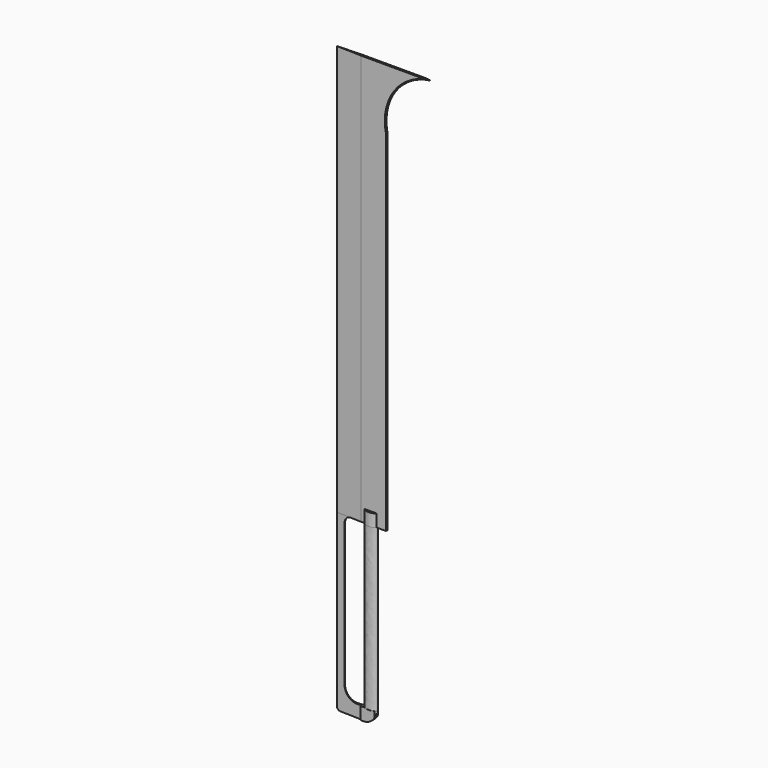
from build123d import *

# Parameters (mm, degrees)
F0_W          = 101.6
F0_H          = 838.2
F1_DEPTH      = 1.905
F3_DEPTH      = 330.2
F3_DEPTH_BACK = 25.4
F5_DEPTH      = 838.201
F7_DEPTH      = 1.905
F9_DEPTH      = 3.96875
F11_DEPTH     = 355.6010001
F13_DEPTH     = 25.401
F14_T2_ANGLE  = 126.8514429449
F14_T4_ANGLE  = 126.8514429449


# Not quite as in the source:
# - a fillet or chamfer that OpenCascade refuses, or shapes differently, is made with other operations: its cross-section is extruded or revolved along the edge and cut away or added


with BuildPart() as f1:
    # F0 (on Front) → F1 (new body, symmetric)
    with BuildSketch(Plane.XZ):
        with Locations((0, 419.1)):
            Rectangle(F0_W, F0_H)
    extrude(amount=F1_DEPTH, both=True)

    # F4 (on face) → F5 (cut, through all)
    with BuildSketch(Plane(origin=(0, 0, 0), x_dir=(1, 0, 0), z_dir=(0, 0, -1))):
        Polygon((-50.8, 0), (0, 1.905), (0, 25.9346883851), (-64.6571069956, 25.9346883851), (-64.6571069956, -15.2188915652), (0, -15.2188915652), (0, -1.905), align=None)
    extrude(amount=-F5_DEPTH, mode=Mode.SUBTRACT)

    # F6 (on Front) → F7 (join, symmetric)
    with BuildSketch(Plane.XZ):
        with BuildLine():
            Line((152.4, 838.2), (50.8, 838.2))
            Line((50.8, 838.2), (50.8, 736.6))
            ThreePointArc((50.8, 736.6), (80.5579510314, 808.4420489686), (152.4, 838.2))
        make_face()
    extrude(amount=F7_DEPTH, both=True)

    # F8 (on Front) → F9 (join, symmetric)
    with BuildSketch(Plane.XZ):
        with BuildLine():
            ThreePointArc((-34.925, -13.0038693017), (-30.7548566659, -3.7760019307), (-21.3588234037, 0))
            add(Edge.make_bspline(
                [(-21.3588234037, 0), (-25.8808822691, 0), (-30.4029411346, 0), (-34.925, 0)],
                knots=[0.420449279, 0.420449279, 0.420449279, 0.420449279, 0.687499999, 0.687499999, 0.687499999, 0.687499999], degree=3))
            add(Edge.make_bspline(
                [(-34.925, 0), (-40.2166666902, 0), (-45.5083333804, 0), (-50.8000000706, 0)],
                knots=[0.687499999, 0.687499999, 0.687499999, 0.687499999, 1, 1, 1, 1], degree=3))
            Line((-50.8000000706, 0), (-50.8000000706, -349.25))
            ThreePointArc((-50.8000000706, -349.25), (-48.9401281311, -353.7401280605), (-44.4500000706, -355.6))
            Line((-44.4500000706, -355.6), (6.35, -355.6))
            ThreePointArc((6.35, -355.6), (24.3105122421, -348.1605122421), (31.75, -330.2))
            Line((31.75, -330.2), (-5.7817636978, -330.2))
            ThreePointArc((-5.7817636978, -330.2), (-26.109357056, -324.3158169798), (-34.925, -305.0773372831))
            Line((-34.925, -305.0773372831), (-34.925, -13.0038693017))
        make_face()
    extrude(amount=F9_DEPTH, both=True)

    # F10 (on face) → F11 (cut, through all)
    with BuildSketch(Plane.XY):
        Polygon((-50.8000000706, -2.6e-09), (0, 1.905), (0, 13.2531421259), (-59.9712096155, 13.2531421259), (-59.9712096155, -14.0750762075), (0, -14.0750762075), (0.0772819473, -1.907898073), align=None)
    extrude(amount=-F11_DEPTH, mode=Mode.SUBTRACT)

    # F12 (on face) → F13 (cut, through all)
    with BuildSketch(Plane.XY.offset(-330.2)):
        with BuildLine():
            add(Edge.make_bspline(
                [(19.05, -6.35), (31.75, -6.35), (31.75, 0), (31.75, 6.35), (19.05, 6.35)],
                knots=[1.5707963268, 1.5707963268, 1.5707963268, 3.1415926536, 3.1415926536, 4.7123889804, 4.7123889804, 4.7123889804], degree=2, weights=[1, 0.7071067812, 1, 0.7071067812, 1]))
            Line((19.05, -6.35), (19.05, -9.2232320458))
            Line((19.05, -9.2232320458), (36.4893190563, -9.2232320458))
            Line((36.4893190563, -9.2232320458), (36.4893190563, 9.4516491517))
            Line((36.4893190563, 9.4516491517), (19.05, 9.4516491517))
            Line((19.05, 9.4516491517), (19.05, 6.35))
        make_face()
    extrude(amount=-F13_DEPTH, mode=Mode.SUBTRACT)

    # F14: chamfer of 2.54 on 2 edges, made by hand

    # F14_s1 → F14_t2 (revolve, cut)
    with BuildSketch(Plane(origin=(-205.6598094156, 0, 617.3107986337), x_dir=(0, 1, 0), z_dir=(0.3160749787, 0, -0.9487342135))):
        Polygon((-1.905, 273.267923448), (0.635, 275.807923448), (-1.905, 275.807923448), align=None)
    revolve(axis=Axis((152.4, -1.905, 736.6), (0, 1, 0)), revolution_arc=F14_T2_ANGLE, mode=Mode.SUBTRACT)

    # F14_s3 → F14_t4 (revolve, cut)
    with BuildSketch(Plane(origin=(-205.6598094156, 0, 617.3107986337), x_dir=(0, 1, 0), z_dir=(0.3160749787, 0, -0.9487342135))):
        Polygon((-0.635, 275.807923448), (1.905, 273.267923448), (1.905, 275.807923448), align=None)
    revolve(axis=Axis((152.4, 1.905, 736.6), (0, 1, 0)), revolution_arc=F14_T4_ANGLE, mode=Mode.SUBTRACT)


with BuildPart() as f3:
    # F2 (on face) → F3 (new body, two sides)
    with BuildSketch(Plane(origin=(0, 0, 0), x_dir=(1, 0, 0), z_dir=(0, 0, -1))) as f3_sk:
        with BuildLine():
            add(Edge.make_bspline(
                [(6.35, 0), (6.35, -10.9985226281), (25.4, -5.499261314), (44.45, 0), (25.4, 5.499261314), (6.35, 10.9985226281), (6.35, 0)],
                knots=[0, 0, 0, 2.0943951024, 2.0943951024, 4.1887902048, 4.1887902048, 6.2831853072, 6.2831853072, 6.2831853072], degree=2, weights=[1, 0.5, 1, 0.5, 1, 0.5, 1]))
        make_face()
    extrude(amount=F3_DEPTH)
    extrude(f3_sk.sketch, amount=-F3_DEPTH_BACK)


solid = Compound([f1.part, f3.part])
